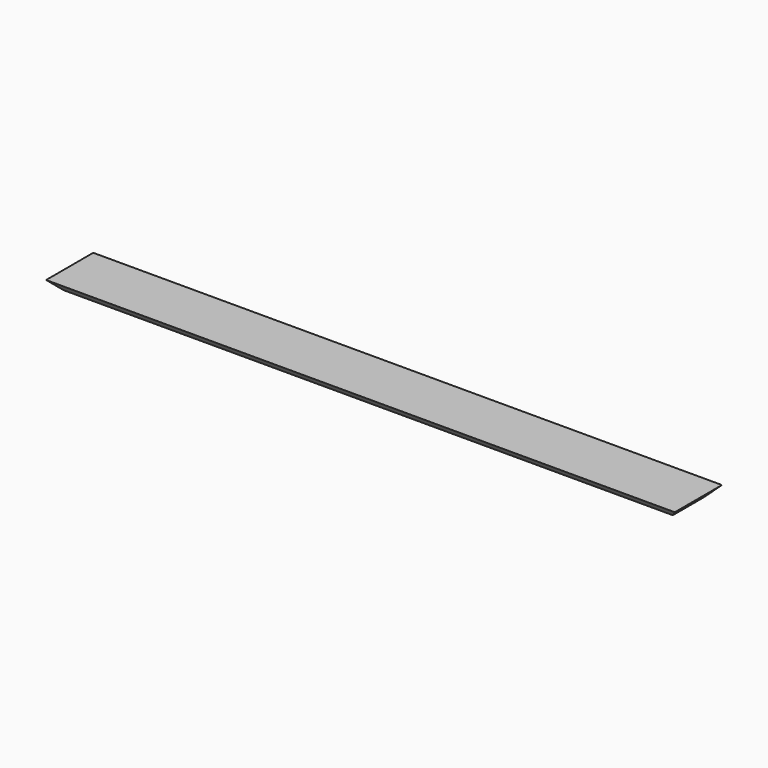
from build123d import *

# Parameters (mm, degrees)
F0_W     = 1600
F0_H     = 150
F1_DEPTH = 12.5
F2_SIZE  = 24.99999


# Not quite as in the source:
# - a fillet or chamfer is up to 0.001 mm smaller than in the source, because OpenCascade refuses the exact size


with BuildPart() as f1:
    # F0 (on Top) → F1 (new body, symmetric)
    with BuildSketch(Plane.XY):
        Rectangle(F0_W, F0_H)
    extrude(amount=F1_DEPTH, both=True)

    # F2 (size 25 in the source; OpenCascade refuses exactly that, so slightly less here)
    f2_edges = [f1.edges().sort_by_distance(p)[0] for p in [
        (0, 75, -12.5),
        (-800, 0, -12.5),
        (0, -75, -12.5),
        (800, 0, -12.5),
    ]]
    chamfer(f2_edges, length=F2_SIZE)


solid = f1.part
